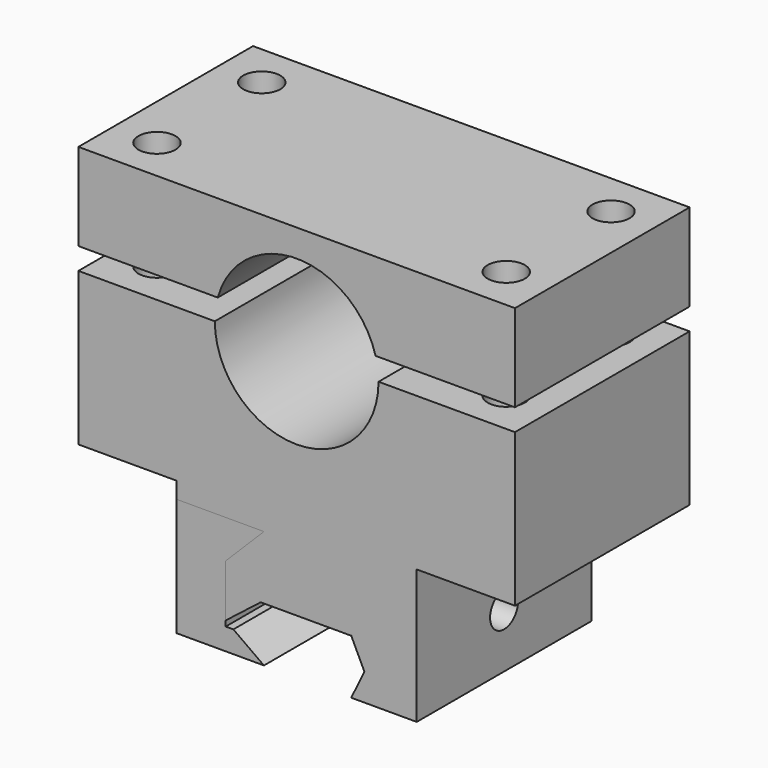
from build123d import *

# Parameters (mm, degrees)
F0_W           = 50.8
F0_H           = 25.4
F1_DEPTH       = 17.78
F3_W           = 50.8
F3_H           = 25.4
F4_DEPTH       = 12.7
F2_R           = 9.525
F5_DEPTH       = 76.2
F6_R           = 9.525
F7_DEPTH       = 76.2
F8_W           = 76.2
F8_H           = 58.4089004228
F9_DEPTH       = 2.54
F10_R          = 2.159
F11_DEPTH      = 17.781
F11_DEPTH_BACK = 25.4
F12_R          = 2.159
F13_DEPTH      = 25.4
F13_DEPTH_BACK = 25.4
F15_DEPTH      = 3.556
F16_W          = 27.94
F16_H          = 12.7
F17_DEPTH      = 1.905
F18_W          = 22.225
F18_H          = 25.4
F19_DEPTH      = 7.366
F22_DEPTH      = 50.8
F23_W          = 22.225
F23_H          = 25.4
F24_DEPTH      = 6.35
F26_DEPTH      = 50.8
F28_DEPTH      = 25.4
F20_R          = 2.032
F29_DEPTH      = 50.8
F29_DEPTH_BACK = 25.4


with BuildPart() as f1:
    # F0 (on Top) → F1 (new body)
    with BuildSketch(Plane.XY):
        Rectangle(F0_W, F0_H)
    extrude(amount=F1_DEPTH)


with BuildPart() as f4:
    # F3 (on face) → F4 (new body)
    with BuildSketch(Plane.XY.offset(17.78)):
        Rectangle(F3_W, F3_H)
    extrude(amount=F4_DEPTH)


with BuildPart() as f5_tool:
    # F2 (on face) → F5 (new body)
    with BuildSketch(Plane.XZ.offset(12.7)):
        with Locations((0, 17.78)):
            Circle(F2_R)
    extrude(amount=-F5_DEPTH)


with BuildPart() as f1_1:
    add(f1.part)

    # F5: cut by f5_tool
    add(f5_tool.part, mode=Mode.SUBTRACT)

    # F6 (on face) → F7 (cut)
    with BuildSketch(Plane.XZ.offset(12.7)):
        with Locations((0, 17.78)):
            Circle(F6_R)
    extrude(amount=-F7_DEPTH, mode=Mode.SUBTRACT)


with BuildPart() as f4_1:
    add(f4.part)

    # F5: cut by f5_tool
    add(f5_tool.part, mode=Mode.SUBTRACT)

    # F8 (on face) → F9 (cut)
    with BuildSketch(Plane(origin=(0, 0, 17.78), x_dir=(1, 0, 0), z_dir=(0, 0, -1))):
        with Locations((12.7, -16.5044502114)):
            Rectangle(F8_W, F8_H)
    extrude(amount=-F9_DEPTH, mode=Mode.SUBTRACT)


with BuildPart() as f11_tool:
    # F10 (on face) → F11 (new body, two sides)
    with BuildSketch(Plane.XY.offset(17.78)) as f11_sk:
        with Locations((-20.32, -7.62)):
            Circle(F10_R)
        with Locations((-20.32, 7.62)):
            Circle(F10_R)
    extrude(amount=-F11_DEPTH)
    extrude(f11_sk.sketch, amount=F11_DEPTH_BACK)


with BuildPart() as f1_2:
    add(f1_1.part)

    # F11: cut by f11_tool
    add(f11_tool.part, mode=Mode.SUBTRACT)


with BuildPart() as f4_2:
    add(f4_1.part)

    # F11: cut by f11_tool
    add(f11_tool.part, mode=Mode.SUBTRACT)


with BuildPart() as f13_tool:
    # F12 (on face) → F13 (new body, two sides)
    with BuildSketch(Plane.XY.offset(17.78)) as f13_sk:
        with Locations((20.32, -7.62)):
            Circle(F12_R)
        with Locations((20.32, 7.62)):
            Circle(F12_R)
    extrude(amount=-F13_DEPTH)
    extrude(f13_sk.sketch, amount=F13_DEPTH_BACK)


with BuildPart() as f1_3:
    add(f1_2.part)

    # F13: cut by f13_tool
    add(f13_tool.part, mode=Mode.SUBTRACT)

    # F14 (on face) → F15 (cut)
    with BuildSketch(Plane(origin=(0, 0, 0), x_dir=(1, 0, 0), z_dir=(0, 0, -1))):
        Polygon((-20.32, 2.794), (-16.1405614013, 5.207), (-16.1405614013, 10.033), (-20.32, 12.446), (-24.4994385987, 10.033), (-24.4994385987, 5.207), align=None)
        Polygon((-16.1405614013, -5.207), (-20.32, -2.794), (-24.4994385987, -5.207), (-24.4994385987, -10.033), (-20.32, -12.446), (-16.1405614013, -10.033), align=None)
        Polygon((16.1405614013, 5.207), (20.32, 2.794), (24.4994385987, 5.207), (24.4994385987, 10.033), (20.32, 12.446), (16.1405614013, 10.033), align=None)
        Polygon((24.4994385987, -10.033), (24.4994385987, -5.207), (20.32, -2.794), (16.1405614013, -5.207), (16.1405614013, -10.033), (20.32, -12.446), align=None)
    extrude(amount=-F15_DEPTH, mode=Mode.SUBTRACT)

    # F16 (on face) → F17 (join)
    with BuildSketch(Plane(origin=(0, 0, 0), x_dir=(1, 0, 0), z_dir=(0, 0, -1))):
        with Locations((0, 6.35)):
            Rectangle(F16_W, F16_H)
        with Locations((0, -6.35)):
            Rectangle(F16_W, F16_H)
    extrude(amount=F17_DEPTH)

    # F18 (on face) → F19 (join)
    with BuildSketch(Plane(origin=(0, 0, -1.905), x_dir=(1, 0, 0), z_dir=(0, 0, -1))):
        with Locations((2.8575, 0)):
            Rectangle(F18_W, F18_H)
    extrude(amount=F19_DEPTH)

    # F21 (on face) → F22 (cut)
    with BuildSketch(Plane(origin=(0, 12.7, 0), x_dir=(-1, 0, 0), z_dir=(0, 1, 0))):
        Polygon((8.255, -6.35), (8.255, -1.905), (3.81, -1.905), align=None)
    extrude(amount=-F22_DEPTH, mode=Mode.SUBTRACT)

    # F23 (on face) → F24 (join)
    with BuildSketch(Plane(origin=(0, 0, -9.271), x_dir=(1, 0, 0), z_dir=(0, 0, -1))):
        with Locations((2.8575, 0)):
            Rectangle(F23_W, F23_H)
    extrude(amount=F24_DEPTH)

    # F25 (on face) → F26 (cut)
    with BuildSketch(Plane(origin=(0, 12.7, 0), x_dir=(-1, 0, 0), z_dir=(0, 1, 0))):
        Polygon((4.191, -9.271), (-6.35, -9.271), (-7.874, -12.446), (-6.35, -15.621), (8.255, -15.621), (8.255, -12.446), align=None)
    extrude(amount=-F26_DEPTH, mode=Mode.SUBTRACT)


with BuildPart() as f4_3:
    add(f4_2.part)

    # F13: cut by f13_tool
    add(f13_tool.part, mode=Mode.SUBTRACT)


with BuildPart() as f28:
    # F27 (on face) → F28 (new body)
    with BuildSketch(Plane.XZ.offset(12.7)):
        Polygon((-3.81, -1.905), (-13.97, -1.905), (-13.97, -13.081), (-8.255, -13.081), (-8.255, -12.446), (-8.255, -6.35), align=None)
        Polygon((-8.255, -13.081), (-13.97, -13.081), (-13.97, -15.621), (-3.81, -15.621), (-7.366, -13.081), align=None)
    extrude(amount=-F28_DEPTH)


with BuildPart() as f29_tool:
    # F20 (on face) → F29 (new body, two sides)
    with BuildSketch(Plane(origin=(-8.255, 0, 0), x_dir=(0, -1, 0), z_dir=(-1, 0, 0))) as f29_sk:
        with Locations((0, -9.271)):
            Circle(F20_R)
    extrude(amount=-F29_DEPTH)
    extrude(f29_sk.sketch, amount=F29_DEPTH_BACK)


with BuildPart() as f1_4:
    add(f1_3.part)

    # F29: cut by f29_tool
    add(f29_tool.part, mode=Mode.SUBTRACT)


with BuildPart() as f28_1:
    add(f28.part)

    # F29: cut by f29_tool
    add(f29_tool.part, mode=Mode.SUBTRACT)


solid = Compound([f4_3.part, f1_4.part, f28_1.part])
